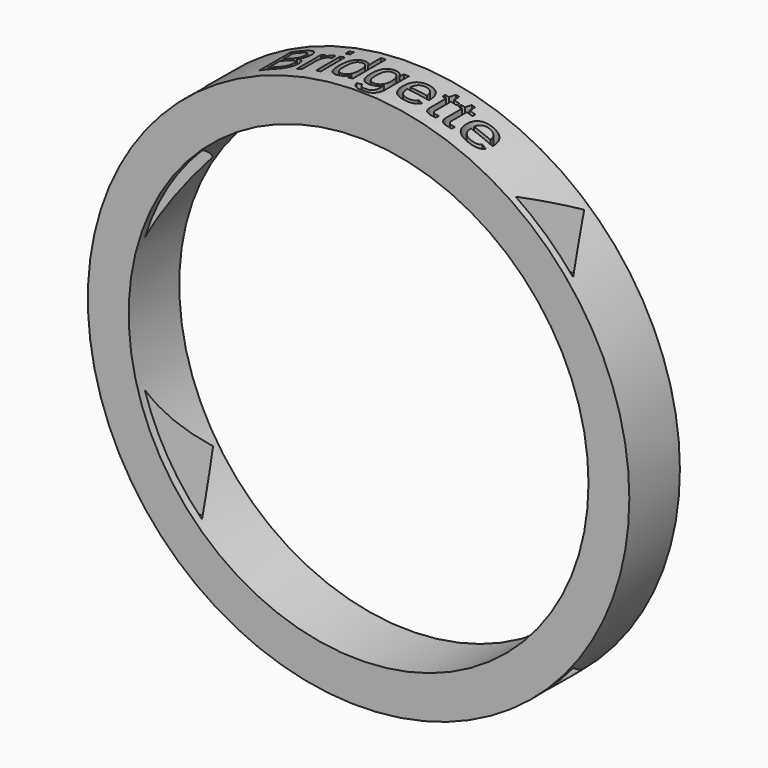
from build123d import *

# Parameters (mm, degrees)
F0_R         = 29.3824116557
F0_R_2       = 24.9492082646
F1_DEPTH     = 6.858
F2_TEXT_SIZE = 6.2119922153
F3_DEPTH     = 52.07
F5_DEPTH     = 25.4
F6_DEPTH     = 25.4


# Not quite as in the source:
# - Text() gives the source's letters only with a copy of the font that has no kerning and outlines rounded to 1/6400 em; it was checked with that copy


with BuildPart() as f1:
    # F0 (on Front) → F1 (new body)
    with BuildSketch(Plane.XZ):
        Circle(F0_R)
        Circle(F0_R_2, mode=Mode.SUBTRACT)
    extrude(amount=F1_DEPTH)

    # F2 (on Top) → F3 (cut)
    with BuildSketch(Plane.XY):
        with Locations((-12.5084286997, -5.3059368402)):
            Text('Bridgette', F2_TEXT_SIZE, font='Arimo', text_align=(TextAlign.LEFT, TextAlign.BOTTOM))
    extrude(amount=F3_DEPTH, mode=Mode.SUBTRACT)

    # F4 (on Top) → F5 (cut)
    with BuildSketch(Plane.XY):
        Polygon((16.4594202111, -6.1197713115), (22.692140304, -6.1197713115), (19.5757802576, -0.7220773763), align=None)
        Polygon((-23.8717740741, -6.0274200514), (-17.6555402577, -6.0274200514), (-20.7636571659, -0.6440036505), align=None)
    extrude(amount=F5_DEPTH, mode=Mode.SUBTRACT)

    # F4 (on Top) → F6 (cut)
    with BuildSketch(Plane.XY):
        Polygon((16.4594202111, -6.1197713115), (22.692140304, -6.1197713115), (19.5757802576, -0.7220773763), align=None)
        Polygon((-23.8717740741, -6.0274200514), (-17.6555402577, -6.0274200514), (-20.7636571659, -0.6440036505), align=None)
    extrude(amount=-F6_DEPTH, mode=Mode.SUBTRACT)


solid = f1.part
